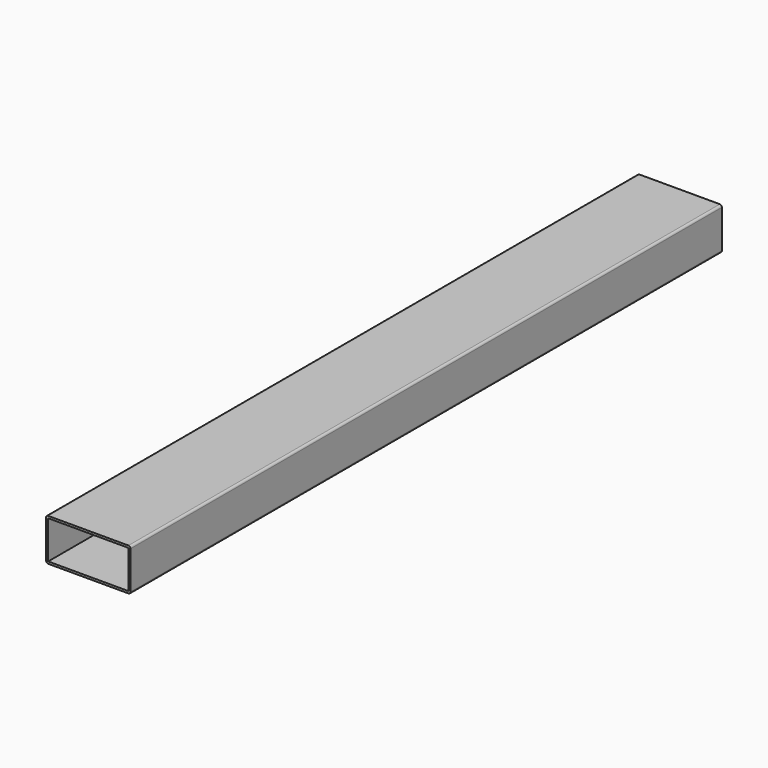
from build123d import *

# Parameters (mm, degrees)
F0_W     = 76
F0_H     = 36
F1_DEPTH = 700


# Not quite as in the source:
# - ends of sketch curves that miss each other by under 0.0002 mm in the source are joined


with BuildPart() as f1:
    # F0 (on Front) → F1 (new body)
    with BuildSketch(Plane.XZ):
        with BuildLine():
            ThreePointArc((-37.999999, 20), (-39.4142135624, 19.4142135624), (-40, 17.999999))
            Line((-40, 17.999999), (-40, -18))
            ThreePointArc((-40, -18), (-39.4142128553, -19.4142142695), (-37.999999, -20))
            Line((-37.999999, -20), (38, -20))
            ThreePointArc((38, -20), (39.4142139159, -19.4142132088), (40, -18))
            Line((40, -18), (40, 18))
            ThreePointArc((40, 18), (39.4142139159, 19.4142132088), (38.000001, 20))
            Line((38.000001, 20), (-37.999999, 20))
        make_face()
        Rectangle(F0_W, F0_H, mode=Mode.SUBTRACT)
    extrude(amount=F1_DEPTH)


solid = f1.part
